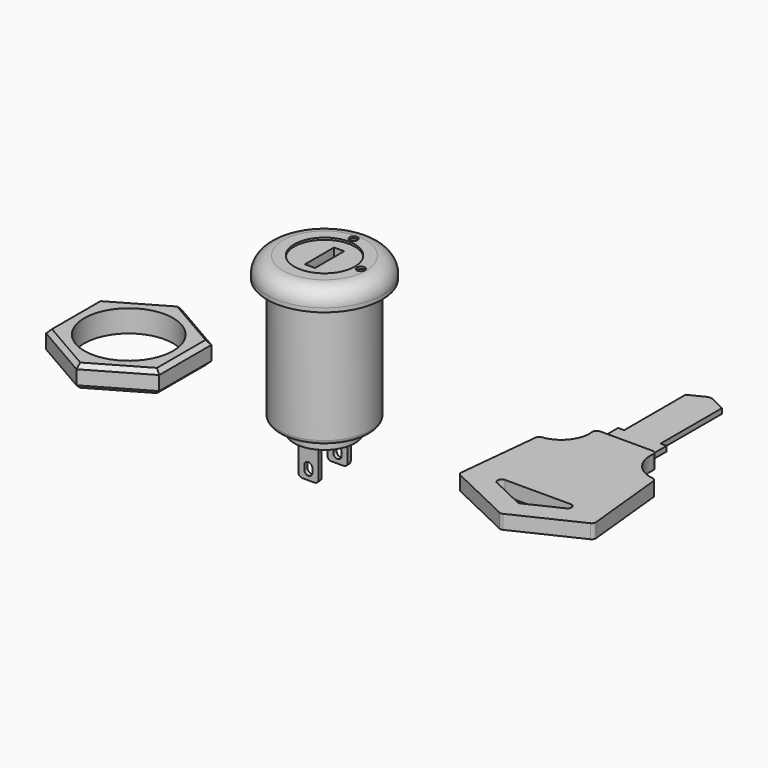
from build123d import *

# Parameters (mm, degrees)
F0_R      = 3.75
F1_DEPTH  = 1.5
F2_START  = 1.5
F0_R_2    = 5.625
F2_DEPTH  = 15.25
F3_START  = 16.75
F0_R_3    = 7.125
F3_DEPTH  = 2.5
F4_DEPTH  = 17.5
F5_W      = 1.25
F5_H      = 4.5
F6_DEPTH  = 10
F5_R      = 0.5
F7_DEPTH  = 0.5
F8_START  = -0.25
F8_DEPTH  = 0.25
F9_W      = 1.25
F9_H      = 0.5
F9_W_2    = 2.5
F10_DEPTH = 0.25
F11_START = 2
F9_H_2    = 3.75
F9_W_3    = 1
F9_H_3    = 1.5
F11_DEPTH = 0.5
F12_START = -2
F12_DEPTH = 0.5
F13_R     = 2
F14_R     = 0.49999
F14_2_R   = 0.49999
F14_3_R   = 0.49999
F15_R     = 5.5
F16_DEPTH = 2.75
F17_SIZE  = 0.5
F19_DEPTH = 0.875
F18_W     = 4.5
F18_H     = 2.5
F18_W_2   = 0.75
F18_H_2   = 10.5
F20_DEPTH = 0.3125
F21_R     = 0.5
F22_SIZE2 = 1
F22_SIZE  = 2


# Not quite as in the source:
# - a fillet or chamfer is up to 0.001 mm smaller than in the source, because OpenCascade refuses the exact size


with BuildPart() as f1:
    # F0 (on Top) → F1 (new body)
    with BuildSketch(Plane.XY):
        Circle(F0_R)
    extrude(amount=F1_DEPTH)


with BuildPart() as f2:
    # F0 (on Top) → F2 (new body)
    with BuildSketch(Plane.XY.offset(F2_START)):
        Circle(F0_R_2)
        Circle(F0_R, mode=Mode.SUBTRACT)
    extrude(amount=F2_DEPTH)

    # F0 (on Top) → F3 (join)
    with BuildSketch(Plane.XY.offset(F3_START)):
        Circle(F0_R_3)
        Circle(F0_R_2, mode=Mode.SUBTRACT)
        Circle(F0_R_2)
        Circle(F0_R, mode=Mode.SUBTRACT)
    extrude(amount=F3_DEPTH)

    # F5 (on face) → F7 (cut)
    with BuildSketch(Plane.XY.offset(19.25)):
        with Locations((0, 4.5)):
            Circle(F5_R)
        with Locations((4.5, 0)):
            Circle(F5_R)
    extrude(amount=-F7_DEPTH, mode=Mode.SUBTRACT)

    # F13
    f13_edges = [f2.edges().sort_by_distance(p)[0] for p in [
        (-7.125, 0, 19.25),
    ]]
    fillet(f13_edges, radius=F13_R)

    # F14#3 (radius 0.5 in the source; OpenCascade refuses exactly that, so slightly less here)
    f14_3_edges = [f2.edges().sort_by_distance(p)[0] for p in [
        (-5.625, 0, 1.5),
    ]]
    fillet(f14_3_edges, radius=F14_3_R)


with BuildPart() as f4:
    # F4 (new, through all): a face of the model
    f4_faces = [f1.part.faces().sort_by_distance(p)[0] for p in [
        (0, 0, 1.5),
    ]]
    extrude(f4_faces, amount=F4_DEPTH)

    # F5 (on face) → F6 (cut)
    with BuildSketch(Plane.XY.offset(19.25)):
        Rectangle(F5_W, F5_H)
    extrude(amount=-F6_DEPTH, mode=Mode.SUBTRACT)


with BuildPart() as f8:
    # F5 (on face) → F8 (new body)
    with BuildSketch(Plane.XY.offset(19.25).offset(F8_START)):
        with Locations((0, 4.5)):
            Circle(F5_R)
    extrude(amount=-F8_DEPTH)


with BuildPart() as f8b:
    # F5 (on face) → F8, piece 2 (new body)
    with BuildSketch(Plane.XY.offset(19.25).offset(F8_START)):
        with Locations((4.5, 0)):
            Circle(F5_R)
    extrude(amount=-F8_DEPTH)


with BuildPart() as f1_1:
    add(f1.part)

    # F9 (on Front) → F10 (join, symmetric)
    with BuildSketch(Plane.XZ):
        with Locations((-1.875, -0.25)):
            Rectangle(F9_W, F9_H)
        with Locations((0, -0.25)):
            Rectangle(F9_W_2, F9_H)
        with Locations((1.875, -0.25)):
            Rectangle(F9_W, F9_H)
    extrude(amount=F10_DEPTH, both=True)


with BuildPart() as f11:
    # F9 (on Front) → F11 (new body)
    with BuildSketch(Plane.XZ.offset(F11_START)):
        with Locations((0, -2.375)):
            Rectangle(F9_W_2, F9_H_2)
        with Locations((0, -3)):
            Rectangle(F9_W_3, F9_H_3, mode=Mode.SUBTRACT)
        with Locations((0, -0.25)):
            Rectangle(F9_W_2, F9_H)
    extrude(amount=F11_DEPTH)

    # F14#2 (radius 0.5 in the source; OpenCascade refuses exactly that, so slightly less here)
    f14_2_edges = [f11.edges().sort_by_distance(p)[0] for p in [
        (1.25, -2.25, -4.25),
        (-1.25, -2.25, -4.25),
        (-0.5, -2.25, -2.25),
        (0.5, -2.25, -2.25),
        (0.5, -2.25, -3.75),
        (-0.5, -2.25, -3.75),
    ]]
    fillet(f14_2_edges, radius=F14_2_R)


with BuildPart() as f12:
    # F9 (on Front) → F12 (new body)
    with BuildSketch(Plane.XZ.offset(F12_START)):
        with Locations((0, -2.375)):
            Rectangle(F9_W_2, F9_H_2)
        with Locations((0, -3)):
            Rectangle(F9_W_3, F9_H_3, mode=Mode.SUBTRACT)
        with Locations((0, -0.25)):
            Rectangle(F9_W_2, F9_H)
    extrude(amount=-F12_DEPTH)

    # F14 (radius 0.5 in the source; OpenCascade refuses exactly that, so slightly less here)
    f14_edges = [f12.edges().sort_by_distance(p)[0] for p in [
        (1.25, 2.25, -4.25),
        (-1.25, 2.25, -4.25),
        (-0.5, 2.25, -2.25),
        (0.5, 2.25, -2.25),
        (0.5, 2.25, -3.75),
        (-0.5, 2.25, -3.75),
    ]]
    fillet(f14_edges, radius=F14_R)


with BuildPart() as f16:
    # F15 (on Top) → F16 (new body)
    with BuildSketch(Plane.XY):
        Polygon((-31.2399982514, 4.0414518843), (-31.2399982514, -4.0414518843), (-24.2399982514, -8.0829037687), (-17.2399982514, -4.0414518843), (-17.2399982514, 4.0414518843), (-24.2399982514, 8.0829037687), align=None)
        with Locations((-24.2399982514, 0)):
            Circle(F15_R, mode=Mode.SUBTRACT)
    extrude(amount=F16_DEPTH)

    # F17
    f17_edges = [f16.edges().sort_by_distance(p)[0] for p in [
        (-20.739998, -6.062178, 2.75),
        (-27.739998, -6.062178, 2.75),
        (-31.239998, 0, 2.75),
        (-27.739998, 6.062178, 2.75),
        (-20.739998, 6.062178, 2.75),
        (-17.239998, 0, 2.75),
        (-20.739998, 6.062178, 0),
        (-27.739998, 6.062178, 0),
        (-31.239998, 0, 0),
        (-27.739998, -6.062178, 0),
        (-20.739998, -6.062178, 0),
        (-17.239998, 0, 0),
    ]]
    chamfer(f17_edges, length=F17_SIZE)


with BuildPart() as f19:
    # F18 (on Top) → F19 (new body, symmetric)
    with BuildSketch(Plane.XY):
        with BuildLine():
            Line((17.75, 10.9423203664), (16.625, 0))
            Line((16.625, 0), (25, -4))
            Line((25, -4), (33.375, 0))
            Line((33.375, 0), (32.25, 10.9423203664))
            ThreePointArc((32.25, 10.9423203664), (29.4375, 12.3485703664), (28.875, 15.4423203664))
            Line((28.875, 15.4423203664), (28, 15.4423203664))
            Line((28, 15.4423203664), (27.25, 15.4423203664))
            Line((27.25, 15.4423203664), (22.75, 15.4423203664))
            Line((22.75, 15.4423203664), (22, 15.4423203664))
            Line((22, 15.4423203664), (21.125, 15.4423203664))
            ThreePointArc((21.125, 15.4423203664), (20.5625, 12.3485703664), (17.75, 10.9423203664))
        make_face()
        Polygon((31.28125, 1.7705066837), (25, -1.2294933163), (18.71875, 1.7705066837), align=None, mode=Mode.SUBTRACT)
    extrude(amount=F19_DEPTH, both=True)

    # F21
    f21_edges = [f19.edges().sort_by_distance(p)[0] for p in [
        (18.71875, 1.770507, 0),
        (25, -1.229493, 0),
        (31.28125, 1.770507, 0),
        (33.375, 0, 0),
        (25, -4, 0),
        (16.625, 0, 0),
        (32.25, 10.94232, 0),
        (28.875, 15.44232, 0),
        (21.125, 15.44232, 0),
        (17.75, 10.94232, 0),
    ]]
    fillet(f21_edges, radius=F21_R)


with BuildPart() as f20:
    # F18 (on Top) → F20 (new body, symmetric)
    with BuildSketch(Plane.XY):
        with Locations((25, 16.6923203664)):
            Rectangle(F18_W, F18_H)
        with Locations((27.625, 16.6923203664)):
            Rectangle(F18_W_2, F18_H)
        with Locations((22.375, 16.6923203664)):
            Rectangle(F18_W_2, F18_H)
        with Locations((25, 23.1923203664)):
            Rectangle(F18_W, F18_H_2)
    extrude(amount=F20_DEPTH, both=True)

    # F22
    f22_edges = [f20.edges().sort_by_distance(p)[0] for p in [
        (27.25, 28.44232, 0),
        (22.75, 28.44232, 0),
    ]]
    f22_side = f20.faces().sort_by_distance((25, 28.44232, 0))[0]
    chamfer(f22_edges, length=F22_SIZE, length2=F22_SIZE2, reference=f22_side)


solid = Compound([f2.part, f4.part, f8.part, f8b.part, f1_1.part, f11.part, f12.part, f16.part, f19.part, f20.part])
